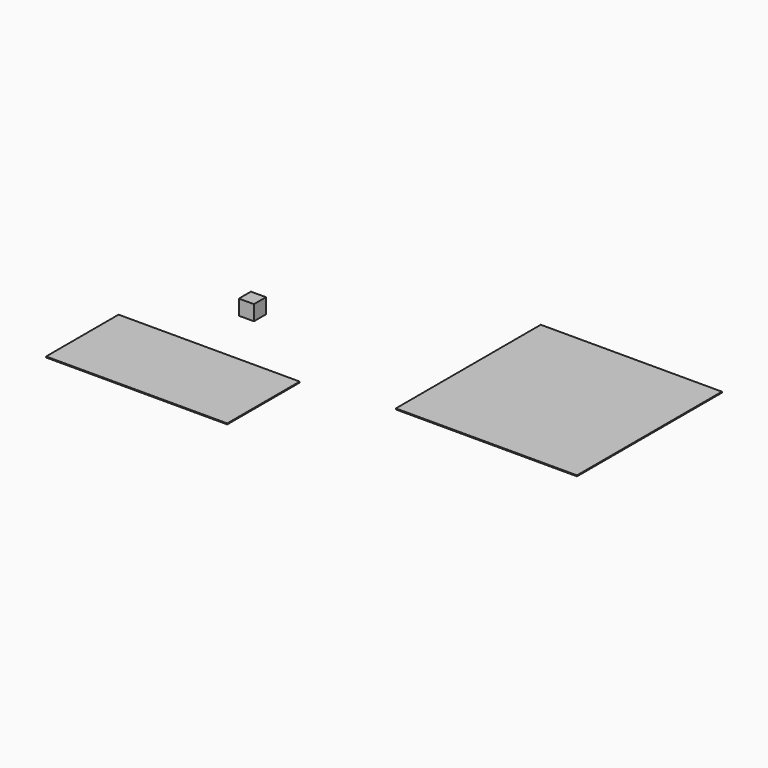
from build123d import *

# Parameters (mm, degrees)
F0_W     = 304.8
F0_H     = 152.4
F1_DEPTH = 1.5875
F2_W     = 304.8
F2_H     = 304.8
F3_DEPTH = 1.5875
F4_W     = 25.4
F4_H     = 25.4
F5_DEPTH = 25.4


# Not quite as in the source:
# - a length typed as a fraction of an inch, garbled in the dataset ("3 / 203.2 mm" for 3/8 in), is restored


with BuildPart() as f1:
    # F0 (on Top) → F1 (new body)
    with BuildSketch(Plane.XY):
        Rectangle(F0_W, F0_H)
    extrude(amount=F1_DEPTH)


with BuildPart() as f3:
    # F2 (on Top) → F3 (new body)
    with BuildSketch(Plane.XY):
        with Locations((451.110124588, 247.8200285587)):
            Rectangle(F2_W, F2_H)
    extrude(amount=F3_DEPTH)


with BuildPart() as f5:
    # F4 (on Right) → F5 (new body)
    with BuildSketch(Plane.YZ):
        with Locations((151.3509980978, 36.8112660944)):
            Rectangle(F4_W, F4_H)
    extrude(amount=F5_DEPTH)


solid = Compound([f1.part, f3.part, f5.part])
